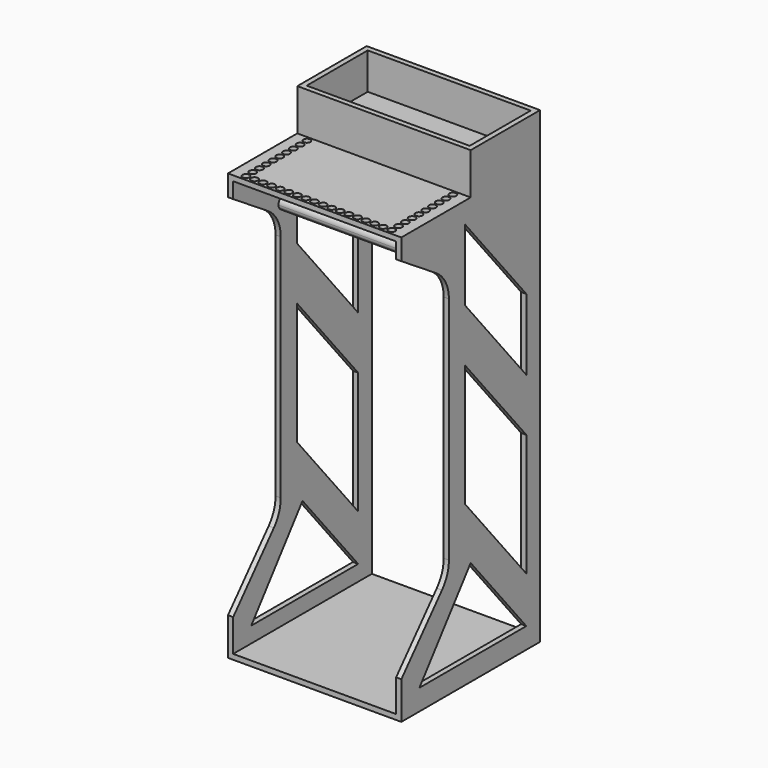
from build123d import *

# Parameters (mm, degrees)
F0_W      = 500
F0_H      = 500
F1_DEPTH  = 15
F2_W      = 15
F2_H      = 500
F3_DEPTH  = 1200
F5_DEPTH  = 500
F6_W      = 500
F6_H      = 500
F7_DEPTH  = 15
F8_W      = 500
F8_H      = 250
F9_DEPTH  = 120
F10_W     = 470
F10_H     = 220
F11_DEPTH = 105
F12_R     = 10
F13_DEPTH = 25
F15_DEPTH = 25
F17_DEPTH = 25
F19_DEPTH = 500


with BuildPart() as f1:
    # F0 (on Top) → F1 (new body)
    with BuildSketch(Plane.XY):
        Rectangle(F0_W, F0_H)
    extrude(amount=F1_DEPTH)

    # F2 (on face) → F3 (join)
    with BuildSketch(Plane.XY.offset(15)):
        with Locations((-242.5, 0)):
            Rectangle(F2_W, F2_H)
        with Locations((242.5, 0)):
            Rectangle(F2_W, F2_H)
    extrude(amount=F3_DEPTH)

    # F4 (on face) → F5 (cut)
    with BuildSketch(Plane(origin=(-250, 0, 0), x_dir=(0, -1, 0), z_dir=(-1, 0, 0))):
        with BuildLine():
            Line((250, 108.3225146088), (250, 1169.652935098))
            Line((250, 1169.652935098), (124.1641795165, 1088.1852527777))
            ThreePointArc((124.1641795165, 1088.1852527777), (90.6620527914, 1052.0193626432), (78.5102322698, 1004.241780428))
            Line((78.5102322698, 1004.241780428), (78.5102322698, 341.1126717917))
            ThreePointArc((78.5102322698, 341.1126717917), (84.9402448732, 305.8329685815), (103.4033814418, 275.090244097))
            Line((103.4033814418, 275.090244097), (250, 108.3225146088))
        make_face()
    extrude(amount=-F5_DEPTH, mode=Mode.SUBTRACT)

    # F6 (on face) → F7 (join)
    with BuildSketch(Plane.XY.offset(1215)):
        Rectangle(F6_W, F6_H)
    extrude(amount=F7_DEPTH)

    # F8 (on face) → F9 (join)
    with BuildSketch(Plane.XY.offset(1230)):
        with Locations((0, 125)):
            Rectangle(F8_W, F8_H)
    extrude(amount=F9_DEPTH)

    # F10 (on face) → F11 (cut)
    with BuildSketch(Plane.XY.offset(1350)):
        with Locations((0, 125)):
            Rectangle(F10_W, F10_H)
    extrude(amount=-F11_DEPTH, mode=Mode.SUBTRACT)

    # F12 (on face) → F13 (cut)
    with BuildSketch(Plane.XY.offset(1230)):
        with Locations((-210.25, -235)):
            Circle(F12_R)
        with Locations((-185.5, -235)):
            Circle(F12_R)
        with Locations((-160.75, -235)):
            Circle(F12_R)
        with Locations((-136, -235)):
            Circle(F12_R)
        with Locations((-111.25, -235)):
            Circle(F12_R)
        with Locations((-86.5, -235)):
            Circle(F12_R)
        with Locations((-61.75, -235)):
            Circle(F12_R)
        with Locations((-37, -235)):
            Circle(F12_R)
        with Locations((-12.25, -235)):
            Circle(F12_R)
        with Locations((12.5, -235)):
            Circle(F12_R)
        with Locations((37.25, -235)):
            Circle(F12_R)
        with Locations((62, -235)):
            Circle(F12_R)
        with Locations((86.75, -235)):
            Circle(F12_R)
        with Locations((111.5, -235)):
            Circle(F12_R)
        with Locations((136.25, -235)):
            Circle(F12_R)
        with Locations((161, -235)):
            Circle(F12_R)
        with Locations((185.75, -235)):
            Circle(F12_R)
        with Locations((210.5, -235)):
            Circle(F12_R)
        with Locations((-210.2958800694, -210.5000429588)):
            Circle(F12_R)
        with Locations((-210.3417601387, -186.0000859177)):
            Circle(F12_R)
        with Locations((-210.3876402081, -161.5001288765)):
            Circle(F12_R)
        with Locations((-210.4335202775, -137.0001718353)):
            Circle(F12_R)
        with Locations((-210.4794003468, -112.5002147941)):
            Circle(F12_R)
        with Locations((-210.5252804162, -88.000257753)):
            Circle(F12_R)
        with Locations((-210.5711604856, -63.5003007118)):
            Circle(F12_R)
        with Locations((-210.6170405549, -39.0003436706)):
            Circle(F12_R)
        with Locations((-210.6629206243, -14.5003866295)):
            Circle(F12_R)
        with Locations((210.4541199306, -210.5000429588)):
            Circle(F12_R)
        with Locations((210.4082398613, -186.0000859177)):
            Circle(F12_R)
        with Locations((210.3623597919, -161.5001288765)):
            Circle(F12_R)
        with Locations((210.3164797225, -137.0001718353)):
            Circle(F12_R)
        with Locations((210.2705996532, -112.5002147941)):
            Circle(F12_R)
        with Locations((210.2247195838, -88.000257753)):
            Circle(F12_R)
        with Locations((210.1788395144, -63.5003007118)):
            Circle(F12_R)
        with Locations((210.1329594451, -39.0003436706)):
            Circle(F12_R)
        with Locations((210.0870793757, -14.5003866295)):
            Circle(F12_R)
    extrude(amount=-F13_DEPTH, mode=Mode.SUBTRACT)

    # F14 (on face) → F15 (cut)
    with BuildSketch(Plane(origin=(-250, 0, 0), x_dir=(0, -1, 0), z_dir=(-1, 0, 0))):
        Polygon((0, 301.9825816154), (-200.6096243858, 60.1997859776), (184.8411858082, 60.1997859776), align=None)
        Polygon((-200.6096243858, 545.617259301), (-200.6096243858, 193.3555305004), (20.2688685386, 459.5671825039), (20.2688685386, 811.8289113045), align=None)
        Polygon((-200.6096243858, 903.4412830945), (-200.6096243858, 697.9457139969), (20.2688685386, 964.1573660004), (20.2688685386, 1169.652935098), align=None)
    extrude(amount=-F15_DEPTH, mode=Mode.SUBTRACT)

    # F16 (on face) → F17 (cut)
    with BuildSketch(Plane.YZ.offset(250)):
        Polygon((200.6096243858, 903.4412830945), (-20.2688685386, 1169.652935098), (-20.2688685386, 964.1573660004), (200.6096243858, 697.9457139969), align=None)
        Polygon((200.6096243858, 545.617259301), (-20.2688685386, 811.8289113045), (-20.2688685386, 459.5671825039), (200.6096243858, 193.3555305004), align=None)
        Polygon((200.6096243858, 60.1997859776), (0, 301.9825816154), (-184.8411858082, 60.1997859776), align=None)
    extrude(amount=-F17_DEPTH, mode=Mode.SUBTRACT)

    # F18 (on face) → F19 (join)
    with BuildSketch(Plane(origin=(-250, 0, 0), x_dir=(0, -1, 0), z_dir=(-1, 0, 0))):
        with BuildLine():
            add(Edge.make_bspline(
                [(53.9202547284, 1096.9846327727), (54.7732887858, 1098.0347093312), (55.4434477794, 1099.2897070818), (56.4611232834, 1100.4414988147)],
                knots=[0, 0, 0, 0, 0.0893664626, 0.0893664626, 0.0893664626, 0.0893664626], degree=3))
            ThreePointArc((53.9202547284, 1096.9846327727), (58.7459698854, 1074.3814357408), (81.7806412913, 1076.2777363651))
            add(Edge.make_bspline(
                [(81.7806412913, 1076.2777363651), (82.0130700174, 1076.5925295791), (82.3047431486, 1076.8573193246), (82.629787133, 1077.224659717)],
                knots=[0, 0, 0, 0, 0.0708567707, 0.0708567707, 0.0708567707, 0.0708567707], degree=3))
            ThreePointArc((82.629787133, 1077.224659717), (83.3571621202, 1078.1603319134), (84.0195396019, 1079.1430897184))
            add(Edge.make_bspline(
                [(84.0195396019, 1079.1430897183), (84.4659025247, 1079.8776865412), (84.8451263222, 1080.6456217553), (85.1639807224, 1081.2907218933)],
                knots=[0.1675578427, 0.1675578427, 0.1675578427, 0.1675578427, 0.2655687466, 0.2655687466, 0.2655687466, 0.2655687466], degree=3))
            ThreePointArc((85.1639807224, 1081.2907218933), (86.3005857895, 1084.7786499445), (86.6850861658, 1088.4268923473))
            ThreePointArc((86.6850861658, 1088.4268923473), (79.4162565109, 1102.6245383975), (63.6481543522, 1105.0278678033))
            add(Edge.make_bspline(
                [(60.3427219255, 1103.5286337913), (61.44755319, 1104.15284537), (62.4027767886, 1104.4920782739), (63.6481543522, 1105.0278678033)],
                knots=[0.1854516751, 0.1854516751, 0.1854516751, 0.1854516751, 0.2676496457, 0.2676496457, 0.2676496457, 0.2676496457], degree=3))
            ThreePointArc((60.3427219255, 1103.5286337913), (58.2920050139, 1102.1232708109), (56.4611232834, 1100.4414988147))
        make_face()
        with BuildLine():
            ThreePointArc((56.4611232834, 1100.4414988147), (55.0843545331, 1098.7912238464), (53.9202547284, 1096.9846327727))
            add(Edge.make_bspline(
                [(53.9202547284, 1096.9846327727), (54.7732887858, 1098.0347093312), (55.4434477794, 1099.2897070818), (56.4611232834, 1100.4414988147)],
                knots=[0, 0, 0, 0, 0.0893664626, 0.0893664626, 0.0893664626, 0.0893664626], degree=3))
        make_face()
        with BuildLine():
            add(Edge.make_bspline(
                [(81.7806412913, 1076.2777363651), (82.0130700174, 1076.5925295791), (82.3047431486, 1076.8573193246), (82.629787133, 1077.224659717)],
                knots=[0, 0, 0, 0, 0.0708567707, 0.0708567707, 0.0708567707, 0.0708567707], degree=3))
            ThreePointArc((81.7806412913, 1076.2777363651), (82.2138198073, 1076.7434810433), (82.629787133, 1077.224659717))
        make_face()
        with BuildLine():
            add(Edge.make_bspline(
                [(56.4611232834, 1100.4414988147), (57.5553096742, 1101.6798845617), (59.0512308325, 1102.798962465), (60.3427219255, 1103.5286337913)],
                knots=[0.0893664626, 0.0893664626, 0.0893664626, 0.0893664626, 0.1854516751, 0.1854516751, 0.1854516751, 0.1854516751], degree=3))
            ThreePointArc((56.4611232834, 1100.4414988147), (58.2920050139, 1102.1232708109), (60.3427219255, 1103.5286337913))
        make_face()
        with BuildLine():
            ThreePointArc((63.6481543522, 1105.0278678033), (61.956464969, 1104.3641767958), (60.3427219255, 1103.5286337913))
            add(Edge.make_bspline(
                [(60.3427219255, 1103.5286337913), (61.44755319, 1104.15284537), (62.4027767886, 1104.4920782739), (63.6481543522, 1105.0278678033)],
                knots=[0.1854516751, 0.1854516751, 0.1854516751, 0.1854516751, 0.2676496457, 0.2676496457, 0.2676496457, 0.2676496457], degree=3))
        make_face()
        with BuildLine():
            add(Edge.make_bspline(
                [(84.0195396019, 1079.1430897183), (84.4659025247, 1079.8776865412), (84.8451263222, 1080.6456217553), (85.1639807224, 1081.2907218933)],
                knots=[0.1675578427, 0.1675578427, 0.1675578427, 0.1675578427, 0.2655687466, 0.2655687466, 0.2655687466, 0.2655687466], degree=3))
            ThreePointArc((84.0195396019, 1079.1430897184), (84.6291363023, 1080.1969886188), (85.1639807224, 1081.2907218933))
        make_face()
    extrude(amount=-F19_DEPTH)


solid = f1.part
